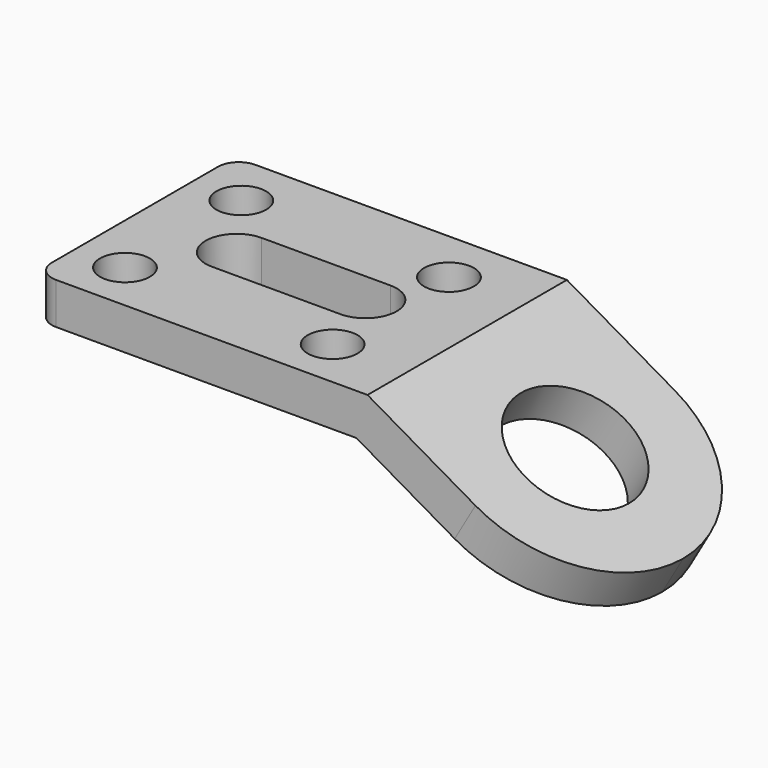
from build123d import *

# Parameters (mm, degrees)
F1_DEPTH = 60
F2_R     = 29.99999
F3_R     = 15
F4_DEPTH = 10
F5_R     = 6
F6_DEPTH = 10
F8_DEPTH = 10
F9_R     = 5


# Not quite as in the source:
# - a fillet or chamfer is up to 0.001 mm smaller than in the source, because OpenCascade refuses the exact size


with BuildPart() as f1:
    # F0 (on Front) → F1 (new body)
    with BuildSketch(Plane.XZ):
        Polygon((80, 0), (0, 0), (0, -10), (77.3205080757, -10), (126.9615242271, -38.6602540378), (131.9615242271, -30), align=None)
    extrude(amount=-F1_DEPTH)

    # F2 (radius 30 in the source; OpenCascade refuses exactly that, so slightly less here)
    f2_edges = [f1.edges().sort_by_distance(p)[0] for p in [
        (129.461524, 0, -34.330127),
        (129.461524, 60, -34.330127),
    ]]
    fillet(f2_edges, radius=F2_R)

    # F3 (on face) → F4 (cut, through all)
    with BuildSketch(Plane(origin=(20, 0, 34.6410161514), x_dir=(0.8660254038, 0, -0.5), z_dir=(0.5, 0, 0.8660254038))):
        with Locations((99.2820323028, 30)):
            Circle(F3_R)
    extrude(amount=-F4_DEPTH, mode=Mode.SUBTRACT)

    # F5 (on face) → F6 (cut, through all)
    with BuildSketch(Plane.XY):
        with Locations((12, 12)):
            Circle(F5_R)
        with Locations((12, 47)):
            Circle(F5_R)
        with Locations((62, 12)):
            Circle(F5_R)
        with Locations((62, 47)):
            Circle(F5_R)
    extrude(amount=-F6_DEPTH, mode=Mode.SUBTRACT)

    # F7 (on face) → F8 (cut, through all)
    with BuildSketch(Plane.XY):
        with BuildLine():
            Line((24.5, 22.5), (55.5, 22.5))
            ThreePointArc((55.5, 22.5), (60.8033008589, 24.6966991411), (63, 30))
            ThreePointArc((63, 30), (60.8033008589, 35.3033008589), (55.5, 37.5))
            Line((55.5, 37.5), (24.5, 37.5))
            ThreePointArc((24.5, 37.5), (19.1966991411, 35.3033008589), (17, 30))
            ThreePointArc((17, 30), (19.1966991411, 24.6966991411), (24.5, 22.5))
        make_face()
    extrude(amount=-F8_DEPTH, mode=Mode.SUBTRACT)

    # F9
    f9_edges = [f1.edges().sort_by_distance(p)[0] for p in [
        (0, 0, -5),
        (0, 60, -5),
    ]]
    fillet(f9_edges, radius=F9_R)


solid = f1.part
